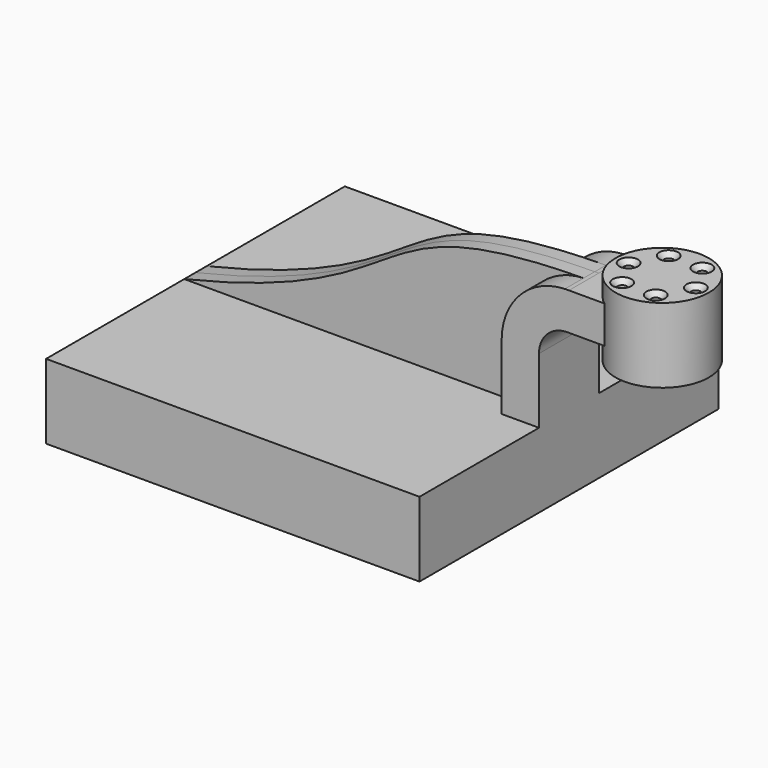
from build123d import *

# Parameters (mm, degrees)
F1_DEPTH        = 100
F0_W            = 25
F0_H            = 20
F2_DEPTH        = 20
F3_DEPTH        = 7.5
F6_D            = 5
F6_CSINK_D      = 10
F6_CSINK_ANGLE  = 90
F6_COPIES_COUNT = 6


# Not quite as in the source:
# - a pattern or mirror of a feature is missing from the dataset's text; its kind, count and spacing are read off the source's solid


with BuildPart() as f1:
    # F0 (on Front) → F1 (new body, symmetric)
    with BuildSketch(Plane.XZ):
        Polygon((-100, -20), (100, -20), (100, 20), (80, 20), (-100, 20), align=None)
    extrude(amount=F1_DEPTH, both=True)

    # F0 (on Front) → F2 (join, symmetric)
    with BuildSketch(Plane.XZ):
        with BuildLine():
            Line((80, 20), (100, 20))
            Line((100, 20), (100, 55))
            ThreePointArc((100, 55), (104.3933982822, 65.6066017178), (115, 70))
            Line((115, 70), (125, 70))
            Line((125, 70), (125, 90))
            Line((125, 90), (116.0234387074, 90))
            add(Edge.make_bspline(
                [(113.8611942755, 89.9814682585), (114.576343668, 89.9888687938), (115.2970695321, 89.9950487976), (116.0234387074, 90)],
                knots=[228.983844188, 228.983844188, 228.983844188, 228.983844188, 230.3162896959, 230.3162896959, 230.3162896959, 230.3162896959], degree=3))
            ThreePointArc((113.8611942755, 89.9814682585), (89.8518569238, 79.3427792132), (80, 55))
            Line((80, 55), (80, 20))
        make_face()
        with Locations((137.5, 80)):
            Rectangle(F0_W, F0_H)
    extrude(amount=F2_DEPTH, both=True)

    # F0 (on Front) → F3 (join, symmetric)
    with BuildSketch(Plane.XZ):
        with BuildLine():
            add(Edge.make_bspline(
                [(-100, 20), (32.7521878521, 51.3916469178), (-9.0388838859, 88.7096691401), (113.8611942755, 89.9814682585)],
                knots=[0, 0, 0, 0, 228.983844188, 228.983844188, 228.983844188, 228.983844188], degree=3))
            Line((-100, 20), (80, 20))
            Line((80, 20), (80, 55))
            ThreePointArc((80, 55), (89.8518569238, 79.3427792132), (113.8611942755, 89.9814682585))
        make_face()
    extrude(amount=F3_DEPTH, both=True)

    # F0 (on Front) → F4 (revolve)
    with BuildSketch(Plane.XZ):
        Polygon((150, 90), (150, 70), (150, 60), (175, 60), (175, 100), (150, 100), align=None)
    revolve(axis=Axis((150, 0, 80), (0, 0, 1)))

    # F6 (through all)
    with Locations(Plane.XY.offset(100)):
        with Locations((168, 0)):
            f6 = CounterSinkHole(F6_D / 2, F6_CSINK_D / 2, counter_sink_angle=F6_CSINK_ANGLE)

    # F6_copies: F6 ×6 about axis
    f6_copies_axis = Axis((150, 0, 0), (0, 0, 1))
    for i in range(1, F6_COPIES_COUNT):
        add(f6.rotate(f6_copies_axis, i * 360 / F6_COPIES_COUNT), mode=Mode.SUBTRACT)


solid = f1.part
